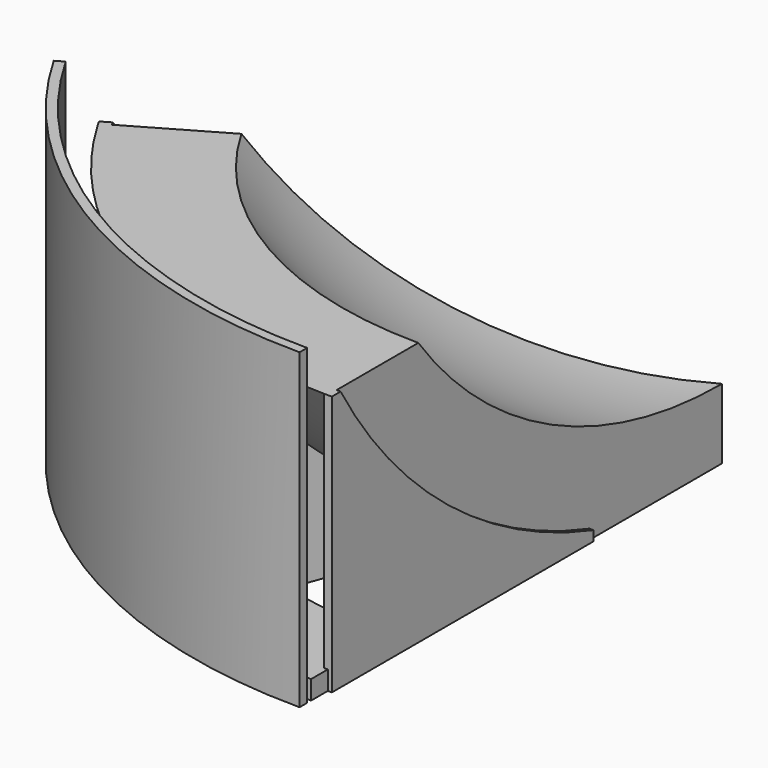
from build123d import *

# Parameters (mm, degrees)
F1_ANGLE = 60
F3_DEPTH = 0.2159
F4_COUNT = 4
F4_ANGLE = 60
F6_DEPTH = 1.016
F8_DEPTH = 16.764


with BuildPart() as f1:
    # F0 (on Right) → F1 (revolve)
    with BuildSketch(Plane.YZ):
        with BuildLine():
            ThreePointArc((0, -25.4), (-11.3875879799, -22.7042471798), (-20.3580009667, -15.1892))
            Line((-20.3580009667, -15.1892), (-26.4257185969, -15.1892))
            ThreePointArc((-26.4257185969, -15.1892), (-18.9823919966, -23.8474148302), (-8.8753284649, -29.1592))
            Line((-8.8753284649, -29.1592), (0, -29.1592))
            Line((0, -29.1592), (0, -25.4))
        make_face()
    revolve(axis=Axis((0, 0, -14.5796), (0, 0, -1)), revolution_arc=F1_ANGLE)



with BuildPart() as f3:
    # F2 (on face) → F3 (new body, symmetric)
    with BuildSketch(Plane.YZ):
        with BuildLine():
            Line((-25.8381304927, -15.1892), (-26.4257185969, -15.1892))
            ThreePointArc((-26.4257185969, -15.1892), (-18.9823919966, -23.8474148302), (-8.8753284649, -29.1592))
            Line((-8.8753284649, -29.1592), (-8.8753284649, -28.6277719818))
            ThreePointArc((-8.8753284649, -28.6277719818), (-18.6119548256, -23.492890873), (-25.8381304927, -15.1892))
        make_face()
        with BuildLine():
            ThreePointArc((-8.8753284649, -29.1592), (-18.9823919966, -23.8474148302), (-26.4257185969, -15.1892))
            Line((-26.4257185969, -15.1892), (-26.4257185969, -29.1592))
            Line((-26.4257185969, -29.1592), (-8.8753284649, -29.1592))
        make_face()
    extrude(amount=F3_DEPTH, both=True)


with BuildPart() as f4_1:
    # F4: instance of F3
    add(f3.part.rotate(Axis((0, 0, -14.5796), (0, 0, -1)), 1 * F4_ANGLE / (F4_COUNT - 1)))


with BuildPart() as f4_2:
    # F4: instance of F3
    add(f3.part.rotate(Axis((0, 0, -14.5796), (0, 0, -1)), 2 * F4_ANGLE / (F4_COUNT - 1)))


with BuildPart() as f4_3:
    # F4: instance of F3
    add(f3.part.rotate(Axis((0, 0, -14.5796), (0, 0, -1)), 3 * F4_ANGLE / (F4_COUNT - 1)))


with BuildPart() as f1_1:
    add(f1.part)

    add(f3.part)  # F6 merges F3

    add(f4_1.part)  # F6 merges F4_1

    add(f4_2.part)  # F6 merges F4_2

    add(f4_3.part)  # F6 merges F4_3
    # F5 (on face) → F6 (join)
    with BuildSketch(Plane(origin=(0, 0, -29.1592), x_dir=(1, 0, 0), z_dir=(0, 0, -1))):
        with BuildLine():
            Line((0, 22.4666516614), (0, 27.5466516614))
            ThreePointArc((0, 27.5466516614), (-13.7817747027, 23.8512201742), (-23.8658510563, 13.7564229039))
            Line((-23.8658510563, 13.7564229039), (-19.4646437932, 11.2195400475))
            ThreePointArc((-19.4646437932, 11.2195400475), (-11.2402166088, 19.4527110569), (0, 22.4666516614))
        make_face()
    extrude(amount=-F6_DEPTH)


with BuildPart() as f8:
    # F7 (on face) → F8 (new body)
    with BuildSketch(Plane(origin=(0, 0, -29.1592), x_dir=(1, 0, 0), z_dir=(0, 0, -1))):
        with BuildLine():
            ThreePointArc((-24.1192543348, 13.8496025107), (-13.9347438766, 24.0701647785), (0, 27.8127654032))
            Line((0, 27.8127654032), (0, 28.3207654032))
            ThreePointArc((0, 28.3207654032), (-14.1892618933, 24.5098061997), (-24.5597923764, 14.1025654208))
            Line((-24.5597923764, 14.1025654208), (-24.1192543348, 13.8496025107))
        make_face()
    extrude(amount=-F8_DEPTH)


solid = Compound([f1_1.part, f8.part])
